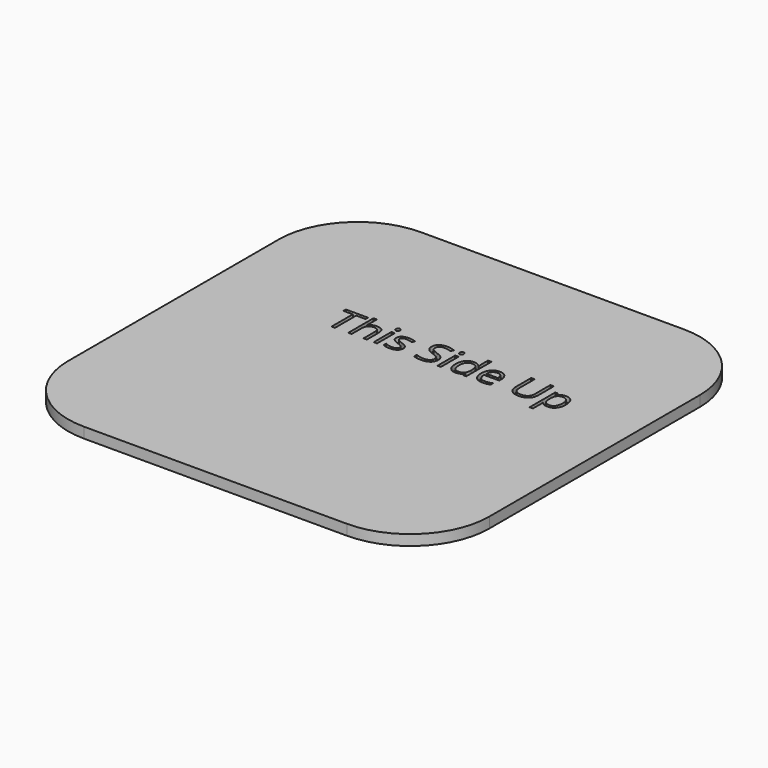
from build123d import *

# Parameters (mm, degrees)
F1_DEPTH     = 2.54
F2_TEXT_SIZE = 9.9932567941
F3_DEPTH     = 1.27


# Not quite as in the source:
# - Text() gives the source's letters only with a copy of the font that has no kerning and outlines rounded to 1/6400 em; it was checked with that copy


with BuildPart() as f1:
    # F0 (on Top) → F1 (new body)
    with BuildSketch(Plane.XY):
        with BuildLine():
            ThreePointArc((50.8, 31.75), (45.2203841816, 45.2203841816), (31.75, 50.8))
            Line((31.75, 50.8), (-31.75, 50.8))
            ThreePointArc((-31.75, 50.8), (-45.2203841816, 45.2203841816), (-50.8, 31.75))
            Line((-50.8, 31.75), (-50.8, -31.75))
            ThreePointArc((-50.8, -31.75), (-45.2203841816, -45.2203841816), (-31.75, -50.8))
            Line((-31.75, -50.8), (31.75, -50.8))
            ThreePointArc((31.75, -50.8), (45.2203841816, -45.2203841816), (50.8, -31.75))
            Line((50.8, -31.75), (50.8, 31.75))
        make_face()
    extrude(amount=F1_DEPTH)

    # F2 (on face) → F3 (cut)
    with BuildSketch(Plane.XY.offset(2.54)):
        with Locations((-23.1683626771, 10.2171041071)):
            Text('This Side Up', F2_TEXT_SIZE, font='Open Sans', text_align=(TextAlign.LEFT, TextAlign.BOTTOM))
    extrude(amount=-F3_DEPTH, mode=Mode.SUBTRACT)


solid = f1.part
